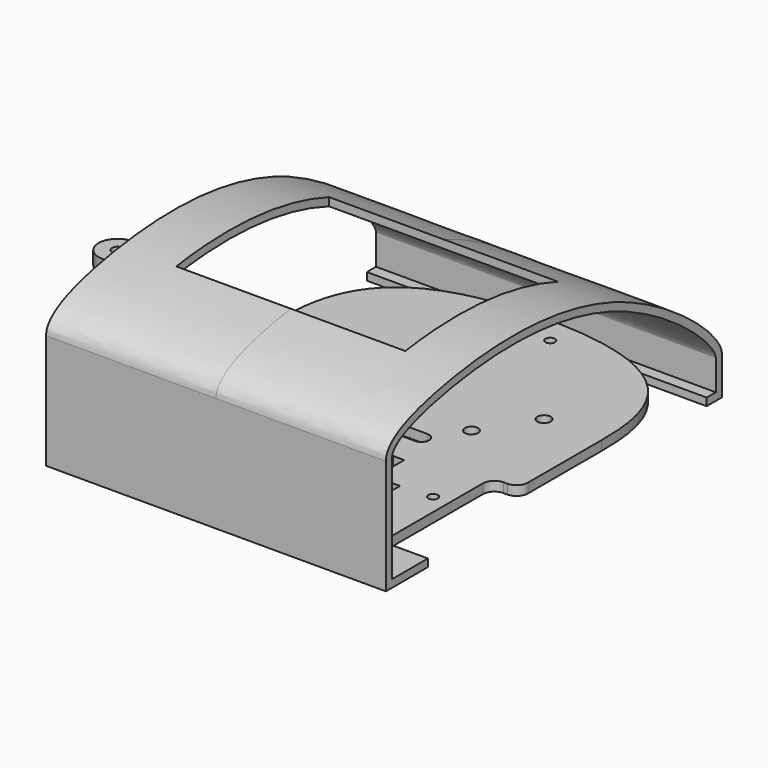
from build123d import *

# Parameters (mm, degrees)
F0_R          = 1.75
F0_R_2        = 1.25
F0_W          = 3
F0_H          = 2
F0_H_2        = 6
F1_DEPTH      = 2.5
F2_R          = 5
F2_R_2        = 1.5
F3_DEPTH      = 3.5
F6_DEPTH      = 44.5
F6_DEPTH_BACK = 44.5
F7_R          = 1.75
F8_DEPTH      = 2
F9_W          = 60
F9_H          = 50
F10_DEPTH     = 228


# Not quite as in the source:
# - an extrude ends at something that could not be found from the text; its depth is read off the source's solid
# - the dataset's text gives a spline's control points without its knots; the knots are read off the source's solid


with BuildPart() as f1:
    # F0 (on Top) → F1 (new body)
    with BuildSketch(Plane.XY):
        with BuildLine():
            Line((4.5, 20), (4.5, 6))
            Line((4.5, 6), (31.5, 6))
            Line((31.5, 6), (31.5, -6))
            Line((31.5, -6), (5.5, -6))
            Line((5.5, -6), (4.5, -6))
            Line((4.5, -6), (4.5, -17))
            ThreePointArc((4.5, -17), (5.3786796564, -19.1213203436), (7.5, -20))
            Line((7.5, -20), (40, -20))
            Line((40, -20), (72.5, -20))
            ThreePointArc((72.5, -20), (74.6213203436, -19.1213203436), (75.5, -17))
            Line((75.5, -17), (75.5, -6))
            Line((75.5, -6), (74.5, -6))
            Line((74.5, -6), (48.5, -6))
            Line((48.5, -6), (48.5, 6))
            Line((48.5, 6), (75.5, 6))
            Line((75.5, 6), (75.5, 20))
            ThreePointArc((75.5, 20), (76.3786796564, 22.1213203436), (78.5, 23))
            Line((78.5, 23), (79.5, 23))
            ThreePointArc((79.5, 23), (81.6213203436, 23.8786796564), (82.5, 26))
            Line((82.5, 26), (82.5, 50))
            add(Edge.make_bspline(
                [(40, 85), (80, 85), (82.5, 65), (82.5, 50)],
                knots=[0, 0, 0, 0, 55.0567888639, 55.0567888639, 55.0567888639, 55.0567888639], degree=3))
            add(Edge.make_bspline(
                [(40, 85), (0, 85), (-2.5, 65), (-2.5, 50)],
                knots=[0, 0, 0, 0, 55.0567888639, 55.0567888639, 55.0567888639, 55.0567888639], degree=3))
            Line((-2.5, 50), (-2.5, 26))
            ThreePointArc((-2.5, 26), (-1.6213203436, 23.8786796564), (0.5, 23))
            Line((0.5, 23), (1.5, 23))
            ThreePointArc((1.5, 23), (3.6213203436, 22.1213203436), (4.5, 20))
        make_face()
        with Locations((15.85, -14)):
            Circle(F0_R, mode=Mode.SUBTRACT)
        with Locations((8.75, -9)):
            Circle(F0_R_2, mode=Mode.SUBTRACT)
        with Locations((18.5, -7.5)):
            Rectangle(F0_W, F0_H, mode=Mode.SUBTRACT)
        with Locations((25, -15)):
            Rectangle(F0_W, F0_H_2, mode=Mode.SUBTRACT)
        with Locations((26.5, -7.5)):
            Rectangle(F0_W, F0_H, mode=Mode.SUBTRACT)
        with Locations((8.75, 9)):
            Circle(F0_R_2, mode=Mode.SUBTRACT)
        with Locations((18.5, 7.5)):
            Rectangle(F0_W, F0_H, mode=Mode.SUBTRACT)
        with Locations((26.5, 7.5)):
            Rectangle(F0_W, F0_H, mode=Mode.SUBTRACT)
        with Locations((25, 15)):
            Rectangle(F0_W, F0_H_2, mode=Mode.SUBTRACT)
        with Locations((55, -15)):
            Rectangle(F0_W, F0_H_2, mode=Mode.SUBTRACT)
        with Locations((53.5, -7.5)):
            Rectangle(F0_W, F0_H, mode=Mode.SUBTRACT)
        with Locations((64.15, -14)):
            Circle(F0_R, mode=Mode.SUBTRACT)
        with Locations((61.5, -7.5)):
            Rectangle(F0_W, F0_H, mode=Mode.SUBTRACT)
        with Locations((71.25, -9)):
            Circle(F0_R_2, mode=Mode.SUBTRACT)
        with Locations((53.5, 7.5)):
            Rectangle(F0_W, F0_H, mode=Mode.SUBTRACT)
        with Locations((55, 15)):
            Rectangle(F0_W, F0_H_2, mode=Mode.SUBTRACT)
        with BuildLine():
            Line((27, 30), (40, 30))
            Line((40, 30), (53, 30))
            ThreePointArc((53, 30), (54.4142135624, 29.4142135624), (55, 28))
            ThreePointArc((55, 28), (54.4142135624, 26.5857864376), (53, 26))
            Line((53, 26), (40, 26))
            Line((40, 26), (27, 26))
            ThreePointArc((27, 26), (25.5857864376, 26.5857864376), (25, 28))
            ThreePointArc((25, 28), (25.5857864376, 29.4142135624), (27, 30))
        make_face(mode=Mode.SUBTRACT)
        with Locations((61.5, 7.5)):
            Rectangle(F0_W, F0_H, mode=Mode.SUBTRACT)
        with Locations((71.25, 9)):
            Circle(F0_R_2, mode=Mode.SUBTRACT)
        with Locations((12.5, 50)):
            Circle(F0_R, mode=Mode.SUBTRACT)
        with Locations((31.15, 36.8)):
            Circle(F0_R, mode=Mode.SUBTRACT)
        with Locations((33.269, 78)):
            Circle(F0_R_2, mode=Mode.SUBTRACT)
        with Locations((59.05, 36.8)):
            Circle(F0_R, mode=Mode.SUBTRACT)
        with Locations((67.5, 50)):
            Circle(F0_R, mode=Mode.SUBTRACT)
        with BuildLine():
            ThreePointArc((12.5, 55), (8.9644660941, 56.4644660941), (7.5, 60))
            Line((7.5, 60), (7.5, 65))
            ThreePointArc((7.5, 65), (8.9644660941, 68.5355339059), (12.5, 70))
            Line((12.5, 70), (40, 70))
            Line((40, 70), (67.5, 70))
            ThreePointArc((67.5, 70), (71.0355339059, 68.5355339059), (72.5, 65))
            Line((72.5, 65), (72.5, 60))
            ThreePointArc((72.5, 60), (71.0355339059, 56.4644660941), (67.5, 55))
            ThreePointArc((67.5, 55), (63.9644660941, 53.5355339059), (62.5, 50))
            ThreePointArc((62.5, 50), (61.9142135624, 48.5857864376), (60.5, 48))
            Line((60.5, 48), (40, 48))
            Line((40, 48), (19.5, 48))
            ThreePointArc((19.5, 48), (18.0857864376, 48.5857864376), (17.5, 50))
            ThreePointArc((17.5, 50), (16.0355339059, 53.5355339059), (12.5, 55))
        make_face(mode=Mode.SUBTRACT)
        with Locations((46.731, 78)):
            Circle(F0_R_2, mode=Mode.SUBTRACT)
        with BuildLine():
            Line((7.5, 65), (7.5, 60))
            ThreePointArc((7.5, 60), (8.9644660941, 56.4644660941), (12.5, 55))
            ThreePointArc((12.5, 55), (16.0355339059, 53.5355339059), (17.5, 50))
            ThreePointArc((17.5, 50), (18.0857864376, 48.5857864376), (19.5, 48))
            Line((19.5, 48), (40, 48))
            Line((40, 48), (60.5, 48))
            ThreePointArc((60.5, 48), (61.9142135624, 48.5857864376), (62.5, 50))
            ThreePointArc((62.5, 50), (63.9644660941, 53.5355339059), (67.5, 55))
            ThreePointArc((67.5, 55), (71.0355339059, 56.4644660941), (72.5, 60))
            Line((72.5, 60), (72.5, 65))
            ThreePointArc((72.5, 65), (71.0355339059, 68.5355339059), (67.5, 70))
            Line((67.5, 70), (40, 70))
            Line((40, 70), (12.5, 70))
            ThreePointArc((12.5, 70), (8.9644660941, 68.5355339059), (7.5, 65))
        make_face()
        Polygon((31.5, 6), (4.5, 6), (4.5, -6), (5.5, -6), (31.5, -6), align=None)
        Polygon((74.5, -6), (75.5, -6), (75.5, 6), (48.5, 6), (48.5, -6), align=None)
    extrude(amount=-F1_DEPTH)


with BuildPart() as f3:
    # F2 (on Top) → F3 (new body)
    with BuildSketch(Plane.XY):
        with Locations((-43.1595407426, 48.7680919468)):
            Circle(F2_R)
        with Locations((-43.1595407426, 48.7680919468)):
            Circle(F2_R_2, mode=Mode.SUBTRACT)
    extrude(amount=F3_DEPTH)


with BuildPart() as f6:
    # F5 (on offset) → F6 (new body, two sides)
    with BuildSketch(Plane.YZ.offset(40)) as f6_sk:
        with BuildLine():
            Line((-12.25, -2.5), (-15.75, -2.5))
            Line((-15.75, -2.5), (-21, -2.5))
            Line((-21, -2.5), (-21, 25.5))
            add(Edge.make_bspline(
                [(-21, 25.5), (-21, 25.5781050911), (-20.9911124841, 25.7288892301), (-20.952660511, 25.948312844), (-20.8874486083, 26.1699194641), (-20.7914832567, 26.4003872849), (-20.6597901353, 26.64344613), (-20.4305125784, 26.9855456903), (-20.033792226, 27.4446825379), (-19.3694209606, 28.0265071996), (-18.5214873984, 28.618527666), (-17.5020148159, 29.2058469221), (-16.3256072333, 29.7787262166), (-15.0072152374, 30.3312111713), (-13.0793861232, 31.0361049017), (-10.9247131131, 31.6893023837), (-8.595814232, 32.2886682663), (-6.7744507078, 32.7116550172), (-4.8907308593, 33.1085671291), (-3.278886914, 33.4181742922), (-1.9703986126, 33.6536070168), (-0.6517979512, 33.8803872049), (1.0156795867, 34.1470874173), (3.0454148554, 34.4383687429), (5.7878431691, 34.7858698253), (9.2791943562, 35.1388617427), (13.5562166224, 35.417116602), (17.9067614491, 35.5349894419), (22.3170127431, 35.4775077822), (26.7732322733, 35.2297726488), (31.2617868122, 34.7769523861), (35.7691768393, 34.1042697735), (40.282068294, 33.1969787314), (44.0364438555, 32.2331079124), (47.0296653103, 31.3299333773), (49.2678502362, 30.584658159), (51.4977251584, 29.7696042711), (53.3477178228, 29.0307344601), (54.8220074929, 28.4027750044), (56.293454008, 27.7499866167), (58.1238908427, 26.8904483549), (60.2972011124, 25.7973380008), (63.1517458539, 24.2686613507), (66.6162430878, 22.2449576248), (70.5355448109, 19.7026984946), (74.1447014078, 17.1143517746), (77.3710849669, 14.5493272365), (79.6790587109, 12.4915515248), (81.2583602323, 10.9332493692), (82.299096667, 9.8200692782), (83.1855361642, 8.775580927), (83.9067291085, 7.8160869046), (84.3608175838, 7.105253498), (84.631647538, 6.6058374731), (84.7882509739, 6.2715372694), (84.899020454, 5.9841865525), (84.9666248098, 5.751912224), (84.997056534, 5.5836927267), (85, 5.5196301955), (85, 5.5)],
                knots=[0, 0, 0, 0, 0.0078125, 0.015625, 0.0234375, 0.03125, 0.0390625, 0.046875, 0.0625, 0.078125, 0.09375, 0.109375, 0.125, 0.140625, 0.15625, 0.1875, 0.203125, 0.21875, 0.234375, 0.25, 0.2578125, 0.265625, 0.28125, 0.296875, 0.3125, 0.34375, 0.375, 0.40625, 0.4375, 0.46875, 0.5, 0.53125, 0.5625, 0.59375, 0.609375, 0.625, 0.640625, 0.65625, 0.6640625, 0.671875, 0.6875, 0.703125, 0.71875, 0.75, 0.78125, 0.8125, 0.84375, 0.875, 0.890625, 0.90625, 0.921875, 0.9375, 0.953125, 0.9609375, 0.96875, 0.9765625, 0.984375, 0.9921875, 1, 1, 1, 1], degree=3))
            Line((85, 5.5), (85, 0))
            Line((85, 0), (85, -2.5))
            Line((85, -2.5), (82, -2.5))
            Line((82, -2.5), (82, -4.5))
            Line((82, -4.5), (87, -4.5))
            Line((87, -4.5), (87, 5.5))
            add(Edge.make_bspline(
                [(-23, 25.5), (-23, 30.5), (1.2676526136, 38.4877659685), (52.843875626, 39.0756277331), (87, 10.5), (87, 5.5)],
                knots=[0, 0, 0, 0, 0.2524532772, 0.6597926628, 1, 1, 1, 1], degree=3))
            Line((-23, 25.5), (-23, -4.5))
            Line((-23, -4.5), (-9.25, -4.5))
            Line((-9.25, -4.5), (-9.25, -2.5))
            Line((-9.25, -2.5), (-12.25, -2.5))
        make_face()
    extrude(amount=F6_DEPTH)
    extrude(f6_sk.sketch, amount=-F6_DEPTH_BACK)

    # F7 (on face) → F8 (cut, through all)
    with BuildSketch(Plane(origin=(0, 0, -4.5), x_dir=(1, 0, 0), z_dir=(0, 0, -1))):
        with Locations((64.15, 14)):
            Circle(F7_R)
        with Locations((15.85, 14)):
            Circle(F7_R)
    extrude(amount=-F8_DEPTH, mode=Mode.SUBTRACT)

    # F9 (on Top) → F10 (cut, through all)
    with BuildSketch(Plane.XY):
        with Locations((40, 26.5)):
            Rectangle(F9_W, F9_H)
    extrude(amount=F10_DEPTH, mode=Mode.SUBTRACT)


solid = Compound([f1.part, f3.part, f6.part])
